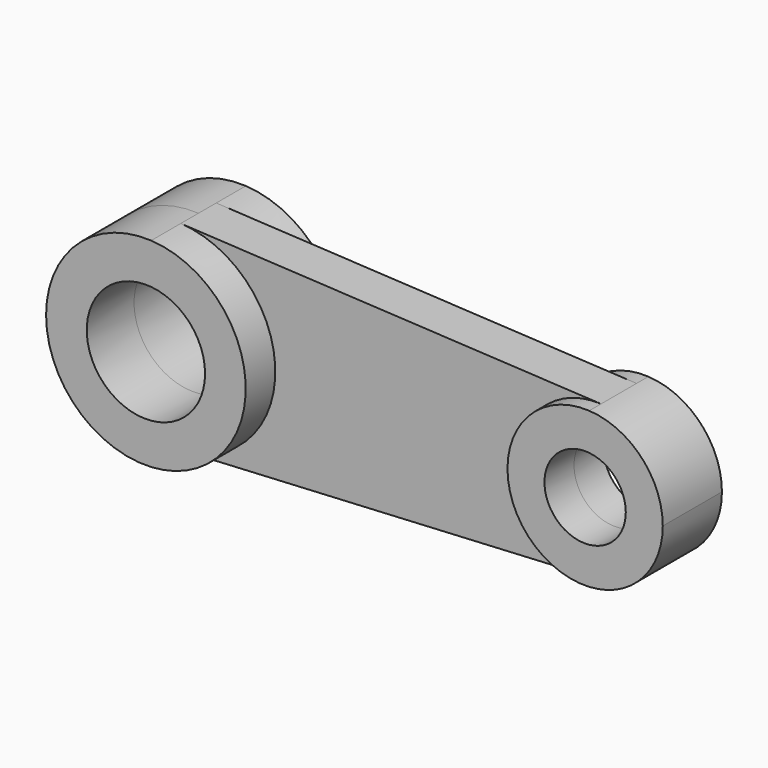
from build123d import *

# Parameters (mm, degrees)
F1_DEPTH = 9.525
F0_R     = 25.4
F2_DEPTH = 25.4
F0_R_2   = 17.4625
F3_DEPTH = 15.875


with BuildPart() as f1:
    # F0 (on Front) → F1 (new body, symmetric)
    with BuildSketch(Plane.XZ):
        with BuildLine():
            ThreePointArc((-23.4888751152, 42.803092487), (5.3509296025, 29.4999956791), (17.1177038322, 0))
            ThreePointArc((17.1177038322, 0), (5.3509296025, -29.4999956791), (-23.4888751152, -42.803092487))
            Line((-23.4888751152, -42.803092487), (156.9848090954, -33.2912941566))
            ThreePointArc((156.9848090954, -33.2912941566), (121.8927038322, 0), (156.9848090954, 33.2912941566))
            Line((156.9848090954, 33.2912941566), (-23.4888751152, 42.803092487))
        make_face()
    extrude(amount=F1_DEPTH, both=True)

    # F0 (on Front) → F2 (join, symmetric)
    with BuildSketch(Plane.XZ):
        with BuildLine():
            ThreePointArc((-23.4888751152, -42.803092487), (5.3509296025, -29.4999956791), (17.1177038322, 0))
            ThreePointArc((17.1177038322, 0), (5.3509296025, 29.4999956791), (-23.4888751152, 42.803092487))
            ThreePointArc((-23.4888751152, 42.803092487), (-68.6072961678, 0), (-23.4888751152, -42.803092487))
        make_face()
        with Locations((-25.7447961678, 0)):
            Circle(F0_R, mode=Mode.SUBTRACT)
    extrude(amount=F2_DEPTH, both=True)

    # F0 (on Front) → F3 (join, symmetric)
    with BuildSketch(Plane.XZ):
        with BuildLine():
            ThreePointArc((188.5677038322, 0), (179.4157683202, 22.9444410837), (156.9848090954, 33.2912941566))
            ThreePointArc((156.9848090954, 33.2912941566), (121.8927038322, 0), (156.9848090954, -33.2912941566))
            ThreePointArc((156.9848090954, -33.2912941566), (179.4157683202, -22.9444410837), (188.5677038322, 0))
        make_face()
        with Locations((155.2302038322, 0)):
            Circle(F0_R_2, mode=Mode.SUBTRACT)
    extrude(amount=F3_DEPTH, both=True)


solid = f1.part
